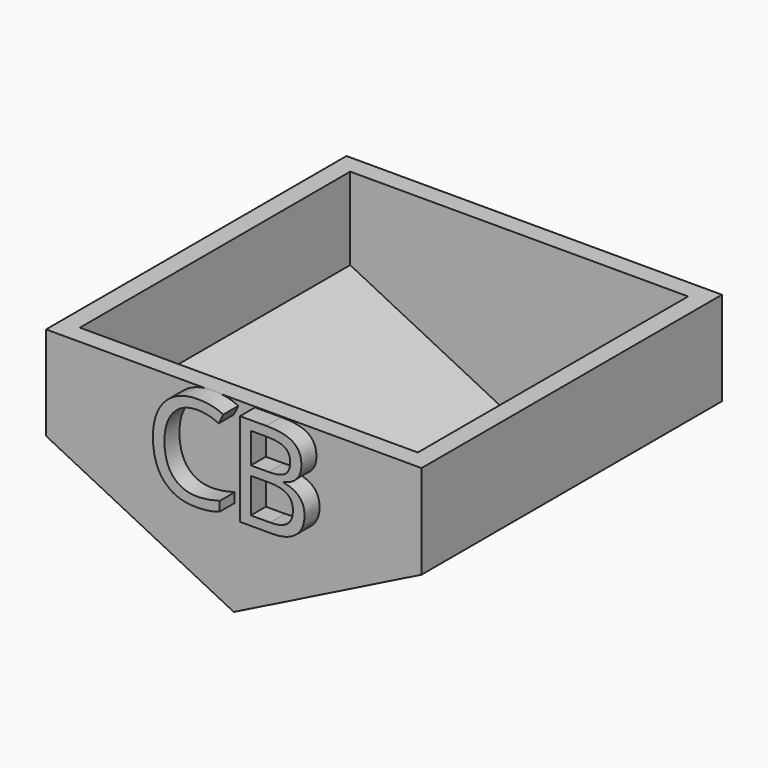
from build123d import *

# Parameters (mm, degrees)
F1_DEPTH     = 50.8
F2_T         = -2.54
F3_TEXT_SIZE = 17.6388888889
F4_DEPTH     = 2.54


# Not quite as in the source:
# - Text() gives the source's letters only with a copy of the font that has no kerning and outlines rounded to 1/6400 em; it was checked with that copy


with BuildPart() as f1:
    # F0 (on Front) → F1 (new body)
    with BuildSketch(Plane.XZ):
        Polygon((0, -12.7), (25.4, 0), (25.4, 12.7), (0, 12.7), align=None)
        Polygon((-25.4, 0), (0, -12.7), (0, 12.7), (-25.4, 12.7), align=None)
    extrude(amount=F1_DEPTH)

    # F2
    f2_openings = [f1.faces().sort_by_distance(p)[0] for p in [
        (0, -25.4, 12.7),
    ]]
    offset(amount=F2_T, openings=f2_openings)

    # F3 (on face) → F4 (join)
    with BuildSketch(Plane.XZ.offset(50.8)):
        with Locations((-9.9920677021, 0)):
            Text('CB', F3_TEXT_SIZE, font='Open Sans', text_align=(TextAlign.LEFT, TextAlign.BOTTOM))
    extrude(amount=F4_DEPTH)


solid = f1.part
